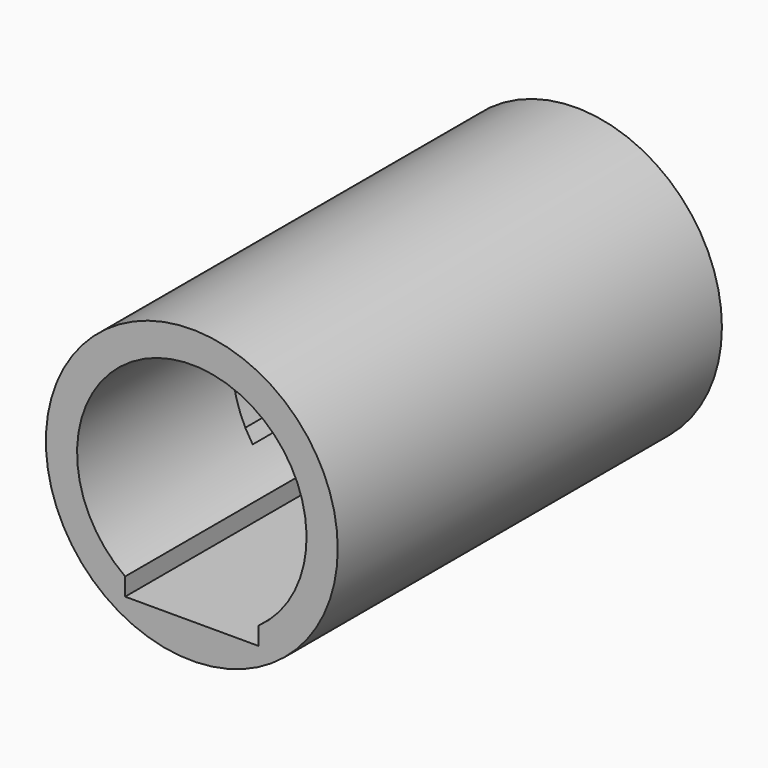
from build123d import *

# Parameters (mm, degrees)
F0_R     = 360.3625
F1_DEPTH = 647.7
F3_DEPTH = 1219.2
F5_W     = 342.9
F5_H     = 393.7
F6_DEPTH = 279.4
F7_R     = 393.7
F7_R_2   = 360.3625
F8_DEPTH = 647.7


# Not quite as in the source:
# - a feature names something its author has since deleted; it is built from what else it names


with BuildPart() as f1:
    # F0 (on Front) → F1 (new body, symmetric)
    with BuildSketch(Plane.XZ):
        Circle(F0_R)
    extrude(amount=F1_DEPTH, both=True)

    # F2 (on face) → F3 (cut)
    with BuildSketch(Plane.XZ.offset(647.7)):
        with BuildLine():
            ThreePointArc((-76.2, -300.0375), (-130.2228778271, -280.8397113954), (-179.7789835799, -252.0088460138))
            Line((-179.7789835799, -252.0088460138), (-179.7789835799, -300.0375))
            Line((-179.7789835799, -300.0375), (-76.2, -300.0375))
        make_face()
        with BuildLine():
            ThreePointArc((179.7685, -252.016324499), (275.2076740277, -141.7380596823), (309.5625, 0))
            ThreePointArc((309.5625, 0), (-141.7323354104, 275.2106220794), (-179.7789835799, -252.0088460138))
            ThreePointArc((-179.7789835799, -252.0088460138), (-130.2228778271, -280.8397113954), (-76.2, -300.0375))
            Line((-76.2, -300.0375), (76.2, -300.0375))
            ThreePointArc((76.2, -300.0375), (130.217036413, -280.8424199334), (179.7685, -252.016324499))
        make_face()
        with BuildLine():
            Line((179.7685, -300.0375), (179.7685, -252.016324499))
            ThreePointArc((179.7685, -252.016324499), (130.217036413, -280.8424199334), (76.2, -300.0375))
            Line((76.2, -300.0375), (179.7685, -300.0375))
        make_face()
    extrude(amount=-F3_DEPTH, mode=Mode.SUBTRACT)

    # F5 (on offset) → F6 (cut)
    with BuildSketch(Plane.YZ.offset(-203.2)):
        with Locations((47.625, 21.0411539862)):
            Rectangle(F5_W, F5_H)
    extrude(amount=-F6_DEPTH, mode=Mode.SUBTRACT)

    # F7 (on Front) → F8 (join, symmetric)
    with BuildSketch(Plane.XZ):
        Circle(F7_R)
        Circle(F7_R_2, mode=Mode.SUBTRACT)
    extrude(amount=F8_DEPTH, both=True)


solid = f1.part
